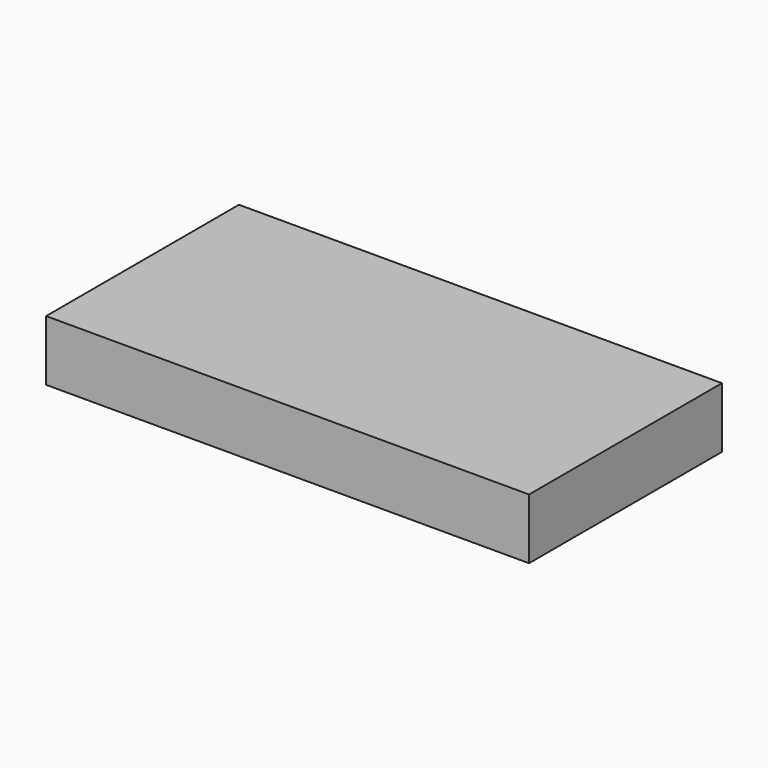
from build123d import *

# Parameters (mm, degrees)
F0_W     = 607.8530848026
F0_H     = 303.4098148346
F1_DEPTH = 76.2


# Not quite as in the source:
# - the program builds the solid bodies; features that only make, move or delete a surface that nothing else refers to are left out


with BuildPart() as f1:
    # F0 (on Top) → F1 (new body)
    with BuildSketch(Plane.XY):
        with Locations((-17.1707123518, 16.9916301966)):
            Rectangle(F0_W, F0_H)
    extrude(amount=F1_DEPTH)


solid = f1.part
